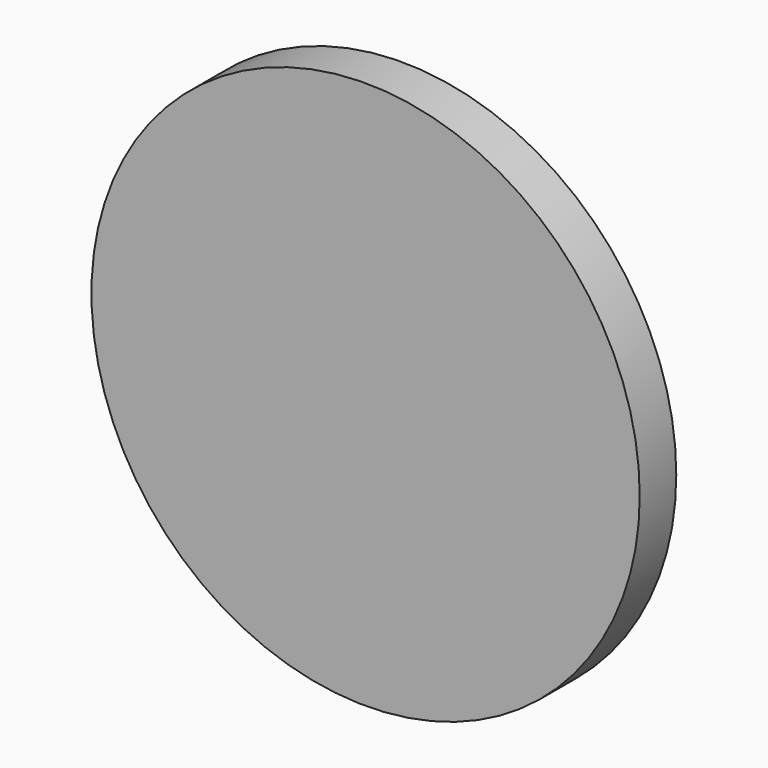
from build123d import *

# Parameters (mm, degrees)
F2_R     = 38.1
F3_DEPTH = 6.35


# Not quite as in the source:
# - the program builds the solid bodies; features that only make, move or delete a surface that nothing else refers to are left out


with BuildPart() as f3:
    # F2 (on Front) → F3 (new body)
    with BuildSketch(Plane.XZ):
        Circle(F2_R)
    extrude(amount=F3_DEPTH)


solid = f3.part
